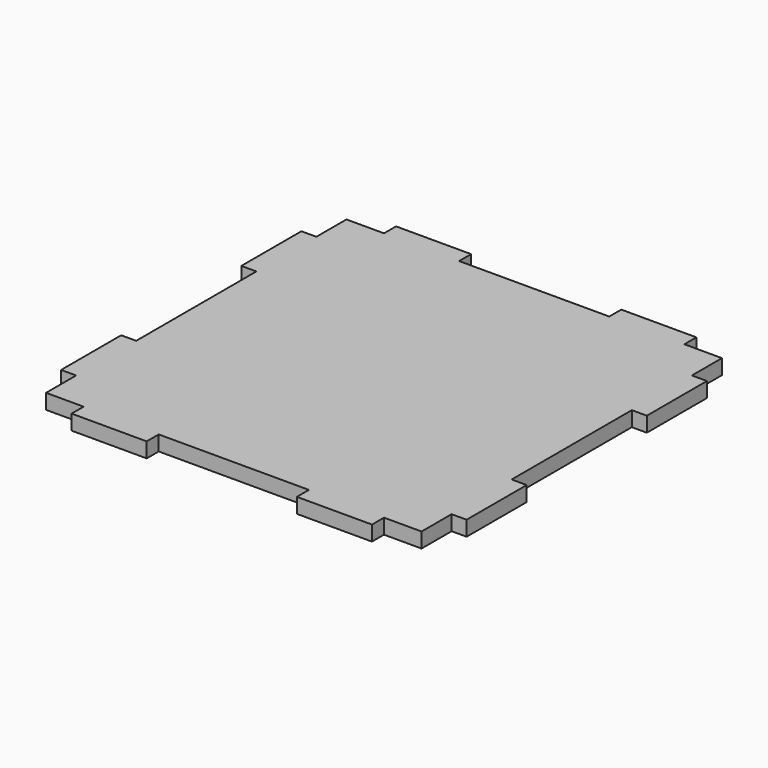
from build123d import *

# Parameters (mm, degrees)
F1_DEPTH = 4


# Not quite as in the source:
# - a feature names something its author has since deleted; it is built from what else it names


with BuildPart() as f1:
    # F0 (on Top) → F1 (new body)
    with BuildSketch(Plane.XY):
        Polygon((50, 40), (50, 50), (40, 50), (40, 54), (20, 54), (20, 50), (-20, 50), (-20, 54), (-40, 54), (-40, 50), (-50, 50), (-50, 40), (-54, 40), (-54, 20), (-50, 20), (-50, -20), (-54, -20), (-54, -40), (-50, -40), (-50, -50), (-40, -50), (-40, -54), (-20, -54), (-20, -50), (20, -50), (20, -54), (40, -54), (40, -50), (50, -50), (50, -40), (54, -40), (54, -20), (50, -20), (50, 20), (54, 20), (54, 40), align=None)
    extrude(amount=F1_DEPTH)


solid = f1.part
